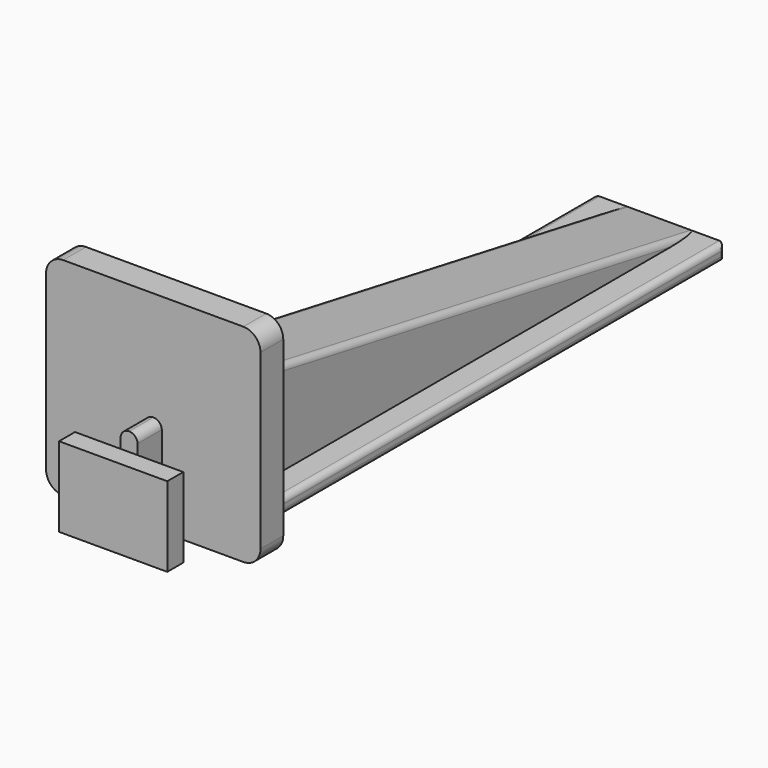
from build123d import *

# Parameters (mm, degrees)
F0_W      = 37.62
F0_H      = 36.35
F1_DEPTH  = 5
F2_W      = 3
F2_H      = 17.2
F3_DEPTH  = 5.3
F4_W      = 19
F4_H      = 14
F5_DEPTH  = 3.5
F6_W      = 23
F6_H      = 22
F7_DEPTH  = 106
F9_DEPTH  = 25
F11_DEPTH = 5
F13_DEPTH = 5
F14_R     = 3
F16_DEPTH = 5.3
F17_R     = 1


with BuildPart() as f1:
    # F0 (on Front) → F1 (new body)
    with BuildSketch(Plane.XZ):
        with Locations((18.81, 18.175)):
            Rectangle(F0_W, F0_H)
    extrude(amount=F1_DEPTH)

    # F2 (on face) → F3 (join)
    with BuildSketch(Plane.XZ.offset(5)):
        with Locations((18.81, 8.6)):
            Rectangle(F2_W, F2_H)
    extrude(amount=F3_DEPTH)

    # F4 (on face) → F5 (join)
    with BuildSketch(Plane.XZ.offset(10.3)):
        with Locations((18.81, 7)):
            Rectangle(F4_W, F4_H)
    extrude(amount=F5_DEPTH)

    # F6 (on face) → F7 (join)
    with BuildSketch(Plane(origin=(0, 0, 0), x_dir=(-1, 0, 0), z_dir=(0, 1, 0))):
        with Locations((-18.81, 11)):
            Rectangle(F6_W, F6_H)
    extrude(amount=F7_DEPTH)

    # F8 (on face) → F9 (cut)
    with BuildSketch(Plane.YZ.offset(30.31)):
        Polygon((106, 22), (0, 22), (106, 2.8), align=None)
    extrude(amount=-F9_DEPTH, mode=Mode.SUBTRACT)

    # F10 (on face) → F11 (cut)
    with BuildSketch(Plane.YZ.offset(30.31)):
        Polygon((0, 2.8), (106, 2.8), (0, 22), align=None)
    extrude(amount=-F11_DEPTH, mode=Mode.SUBTRACT)

    # F12 (on face) → F13 (cut)
    with BuildSketch(Plane(origin=(7.31, 0, 0), x_dir=(0, -1, 0), z_dir=(-1, 0, 0))):
        Polygon((0, 22), (-106, 2.8), (0, 2.8), align=None)
    extrude(amount=-F13_DEPTH, mode=Mode.SUBTRACT)

    # F14
    f14_edges = [f1.edges().sort_by_distance(p)[0] for p in [
        (37.62, -2.5, 0),
        (37.62, -2.5, 36.35),
        (0, -2.5, 36.35),
        (0, -2.5, 0),
    ]]
    fillet(f14_edges, radius=F14_R)

    # F15 (on face) → F16 (cut, through all)
    with BuildSketch(Plane.XZ.offset(10.3)):
        with BuildLine():
            ThreePointArc((17.31, 15.79375), (17.7819509907, 16.79346061), (18.81, 17.2))
            Line((18.81, 17.2), (17.31, 17.2))
            Line((17.31, 17.2), (17.31, 15.79375))
        make_face()
        with BuildLine():
            ThreePointArc((18.81, 17.2), (19.8380490093, 16.79346061), (20.31, 15.79375))
            Line((20.31, 15.79375), (20.31, 17.2))
            Line((20.31, 17.2), (18.81, 17.2))
        make_face()
    extrude(amount=-F16_DEPTH, mode=Mode.SUBTRACT)

    # F17
    f17_edges = [f1.edges().sort_by_distance(p)[0] for p in [
        (30.31, 106, 1.4),
        (7.31, 106, 1.4),
        (7.31, 53, 2.8),
        (7.31, 53, 0),
        (25.31, 53, 12.4),
        (30.31, 53, 2.8),
        (30.31, 53, 0),
        (12.31, 53, 12.4),
    ]]
    fillet(f17_edges, radius=F17_R)


solid = f1.part
